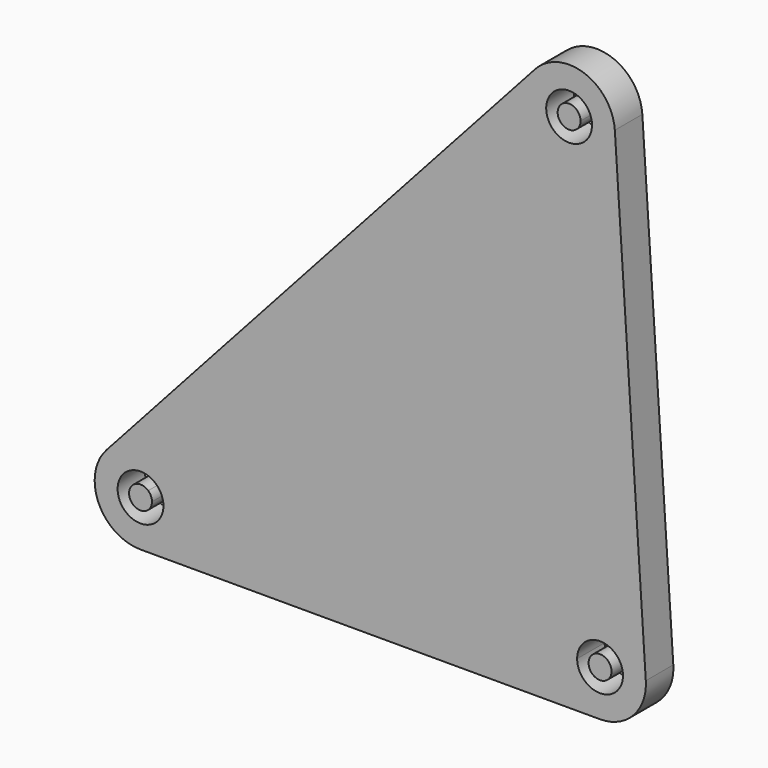
from build123d import *

# Parameters (mm, degrees)
F1_DEPTH = 76.2


# Not quite as in the source:
# - ends of sketch curves that miss each other by under 0.0002 mm in the source are joined


with BuildPart() as f1:
    # F0 (on Front) → F1 (new body)
    with BuildSketch(Plane.XZ):
        with BuildLine():
            Line((874.5321444168, 1119.9607458335), (-75.4025189249, 68.0956794957))
            ThreePointArc((-75.4025189249, 68.0956794957), (-92.8468646719, -41.2555416955), (0, -101.6))
            Line((0, -101.6), (1018.54, -101.6))
            ThreePointArc((1018.54, -101.6), (1092.6830925881, -69.4648243464), (1119.9245847073, 6.6125625695))
            Line((1119.9245847073, 6.6125625695), (1051.3192480489, 1058.4776289074))
            ThreePointArc((1051.3192480489, 1058.4776289074), (983.3084595803, 1147.8272970572), (874.5321444168, 1119.9607458335))
        make_face()
        with BuildLine():
            Line((967.74, 0), (50.8, 0))
            ThreePointArc((50.8, 0), (-46.423432336, -20.6277708478), (34.0478373958, 37.701256858))
            Line((34.0478373958, 37.701256858), (915.8868259459, 1014.1638094799))
            ThreePointArc((915.8868259459, 1014.1638094799), (929.3068924939, 1098.2884986738), (1000.7346633416, 1051.8650663379))
            ThreePointArc((1000.7346633416, 1051.8650663379), (987.0062096357, 1017.1326541647), (953.2409446264, 1001.1727739842))
            Line((953.2409446264, 1001.1727739842), (1015.2337187153, 50.6922923536))
            ThreePointArc((1015.2337187153, 50.6922923536), (1053.2724121732, 37.0715462941), (1069.34, 0))
            ThreePointArc((1069.34, 0), (1018.54, -50.8), (967.74, 0))
        make_face(mode=Mode.SUBTRACT)
        with BuildLine():
            ThreePointArc((34.0478373958, 37.701256858), (46.423432336, 20.6277708478), (50.8, 0))
            Line((50.8, 0), (967.74, 0))
            ThreePointArc((967.74, 0), (981.4684537059, 34.7324121732), (1015.2337187153, 50.6922923536))
            Line((1015.2337187153, 50.6922923536), (953.2409446264, 1001.1727739842))
            ThreePointArc((953.2409446264, 1001.1727739842), (933.2477652223, 1003.8839509782), (915.8868259459, 1014.1638094799))
            Line((915.8868259459, 1014.1638094799), (34.0478373958, 37.701256858))
        make_face()
    extrude(amount=F1_DEPTH)


with BuildPart() as f1b:
    # F0 (on Front) → F1, piece 2 (new body)
    with BuildSketch(Plane.XZ):
        with BuildLine():
            Line((25.4, 0), (0, 0))
            Line((0, 0), (17.0239186979, 18.850628429))
            ThreePointArc((17.0239186979, 18.850628429), (-23.211716168, -10.3138854239), (25.4, 0))
        make_face()
        with BuildLine():
            Line((17.0239186979, 18.850628429), (0, 0))
            Line((0, 0), (25.4, 0))
            ThreePointArc((25.4, 0), (23.211716168, 10.3138854239), (17.0239186979, 18.850628429))
        make_face()
    extrude(amount=F1_DEPTH)


with BuildPart() as f1c:
    # F0 (on Front) → F1, piece 3 (new body)
    with BuildSketch(Plane.XZ):
        with BuildLine():
            Line((1018.54, 0), (993.14, 0))
            ThreePointArc((993.14, 0), (1018.54, -25.4), (1043.94, 0))
            ThreePointArc((1043.94, 0), (1035.9062060866, 18.535773147), (1016.8868593576, 25.3461461768))
            Line((1016.8868593576, 25.3461461768), (1018.54, 0))
        make_face()
        with BuildLine():
            ThreePointArc((1016.8868593576, 25.3461461768), (1000.004226853, 17.3662060866), (993.14, 0))
            Line((993.14, 0), (1018.54, 0))
            Line((1018.54, 0), (1016.8868593576, 25.3461461768))
        make_face()
    extrude(amount=F1_DEPTH)


with BuildPart() as f1d:
    # F0 (on Front) → F1, piece 4 (new body)
    with BuildSketch(Plane.XZ):
        with BuildLine():
            Line((949.9346633416, 1051.8650663379), (932.9107446438, 1033.0144379089))
            ThreePointArc((932.9107446438, 1033.0144379089), (941.591214282, 1027.8745086581), (951.587803984, 1026.5189201611))
            Line((951.587803984, 1026.5189201611), (949.9346633416, 1051.8650663379))
        make_face()
        with BuildLine():
            ThreePointArc((975.3346633416, 1051.8650663379), (939.6207779178, 1075.0767825059), (932.9107446438, 1033.0144379089))
            Line((932.9107446438, 1033.0144379089), (949.9346633416, 1051.8650663379))
            Line((949.9346633416, 1051.8650663379), (951.587803984, 1026.5189201611))
            ThreePointArc((951.587803984, 1026.5189201611), (968.4704364887, 1034.4988602513), (975.3346633416, 1051.8650663379))
        make_face()
    extrude(amount=F1_DEPTH)


solid = Compound([f1.part, f1b.part, f1c.part, f1d.part])
